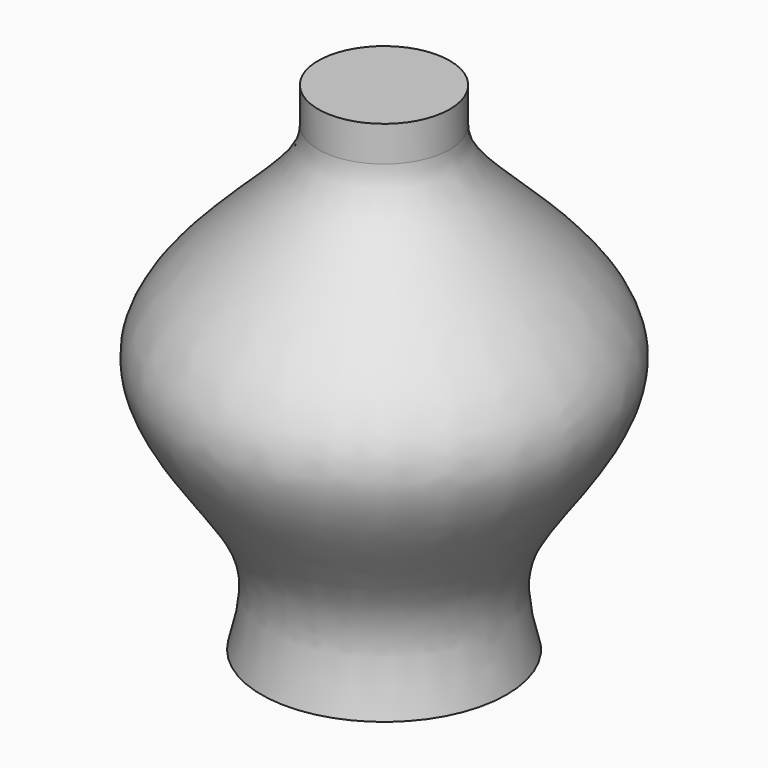
from build123d import *


with BuildPart() as f1:
    # F0 (on Front) → F1 (revolve)
    with BuildSketch(Plane.XZ):
        with BuildLine():
            Line((14.0401206778, 50.1161552966), (0, 50.1161552966))
            Line((0, 50.1161552966), (0, -56.1730787158))
            Line((0, -56.1730787158), (26.1815413833, -55.9776946902))
            add(Edge.make_bspline(
                [(26.1815413833, -55.9776946902), (24.4131565466, -49.2499493412), (20.209988544, -33.2591743733), (61.9659793922, 2.8491265853), (15.4256031143, 30.789337421), (14.0656178298, 41.3113405605), (14.0401206778, 42.5489448246)],
                knots=[0, 0, 0, 0, 0.2091032484, 0.4970049872, 0.8053885573, 0.8605358957, 0.8605358957, 0.8605358957, 0.8605358957], degree=3))
            add(Edge.make_bspline(
                [(14.0401206778, 42.5489448246), (14.036067117, 42.7457002938), (14.0365835548, 42.9333928057), (14.0401206778, 43.111050345)],
                knots=[0.8605358957, 0.8605358957, 0.8605358957, 0.8605358957, 0.8693032705, 0.8693032705, 0.8693032705, 0.8693032705], degree=3))
            Line((14.0401206778, 43.111050345), (14.0401206778, 45.0370277254))
            Line((14.0401206778, 45.0370277254), (14.0401206778, 50.1161552966))
        make_face()
        with BuildLine():
            add(Edge.make_bspline(
                [(14.0401206778, 42.5489448246), (14.036067117, 42.7457002938), (14.0365835548, 42.9333928057), (14.0401206778, 43.111050345)],
                knots=[0.8605358957, 0.8605358957, 0.8605358957, 0.8605358957, 0.8693032705, 0.8693032705, 0.8693032705, 0.8693032705], degree=3))
            Line((14.0401206778, 42.5489448246), (14.0401206778, 43.111050345))
        make_face()
    revolve(axis=Axis((0, 0, -3.0284617096), (0, 0, -1)))


solid = f1.part
